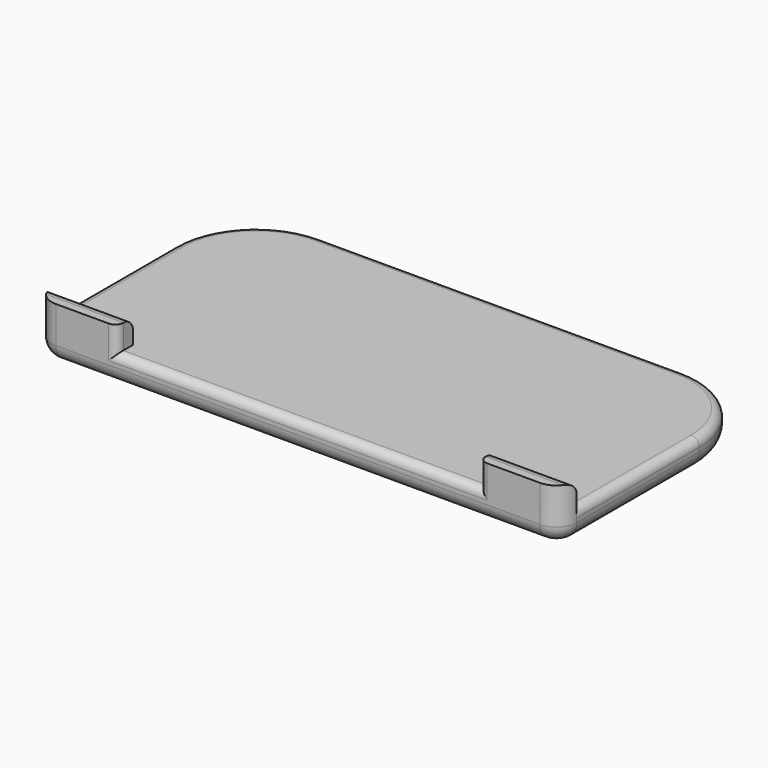
from build123d import *

# Parameters (mm, degrees)
F1_DEPTH    = 8.89
F3_DEPTH    = 7.62
F4_T1_DEPTH = 47.8505725861
F4_T3_DEPTH = 113.1511068404
F4_T6_ANGLE = 90
F4_T8_ANGLE = 90
F5_R        = 5.08
F6_R        = 3.81
F7_R        = 2.54


# Not quite as in the source:
# - a fillet or chamfer that OpenCascade refuses, or shapes differently, is made with other operations: its cross-section is extruded or revolved along the edge and cut away or added


with BuildPart() as f1:
    # F0 (on Top) → F1 (new body)
    with BuildSketch(Plane.XY):
        with BuildLine():
            Line((22.7506106496, 59.7472505152), (-90.4004961908, 59.7472505152))
            ThreePointArc((-90.4004961908, 59.7472505152), (-108.3610084329, 52.3077627574), (-115.8004961908, 34.3472505152))
            Line((-115.8004961908, 34.3472505152), (-115.8004961908, -13.5033220708))
            ThreePointArc((-115.8004961908, -13.5033220708), (-113.9406242513, -17.9934501314), (-109.4504961908, -19.8533220708))
            Line((-109.4504961908, -19.8533220708), (41.8006106496, -19.8533220708))
            ThreePointArc((41.8006106496, -19.8533220708), (46.2907387101, -17.9934501314), (48.1506106496, -13.5033220708))
            Line((48.1506106496, -13.5033220708), (48.1506106496, 34.3472505152))
            ThreePointArc((48.1506106496, 34.3472505152), (40.7111228917, 52.3077627574), (22.7506106496, 59.7472505152))
        make_face()
    extrude(amount=F1_DEPTH)

    # F2 (on face) → F3 (join)
    with BuildSketch(Plane.XY.offset(8.89)):
        with BuildLine():
            ThreePointArc((41.8006106496, -19.8533220708), (46.2907387101, -17.9934501314), (48.1506106496, -13.5033220708))
            Line((48.1506106496, -13.5033220708), (22.7506106496, -13.5033220708))
            Line((22.7506106496, -13.5033220708), (22.7506106496, -19.8533220708))
            Line((22.7506106496, -19.8533220708), (41.8006106496, -19.8533220708))
        make_face()
        with BuildLine():
            Line((-90.4004961908, -13.5033220708), (-115.8004961908, -13.5033220708))
            ThreePointArc((-115.8004961908, -13.5033220708), (-113.9406242513, -17.9934501314), (-109.4504961908, -19.8533220708))
            Line((-109.4504961908, -19.8533220708), (-90.4004961908, -19.8533220708))
            Line((-90.4004961908, -19.8533220708), (-90.4004961908, -13.5033220708))
        make_face()
    extrude(amount=F3_DEPTH)

    # F4: fillet of radius 2.54 on 1 edges, made by hand

    # F4_s2 → F4_t1 (cut)
    with BuildSketch(Plane.XZ.offset(-34.3472505152)):
        with BuildLine():
            ThreePointArc((45.6106106496, 8.89), (47.4066618738, 8.1460512242), (48.1506106496, 6.35))
            Line((48.1506106496, 6.35), (48.1506106496, 8.89))
            Line((48.1506106496, 8.89), (45.6106106496, 8.89))
        make_face()
        with BuildLine():
            ThreePointArc((-113.2604961908, 8.89), (-115.056547415, 8.1460512242), (-115.8004961908, 6.35))
            Line((-115.8004961908, 6.35), (-115.8004961908, 8.89))
            Line((-115.8004961908, 8.89), (-113.2604961908, 8.89))
        make_face()
    extrude(amount=F4_T1_DEPTH, mode=Mode.SUBTRACT)

    # F4_s4 → F4_t3 (cut)
    with BuildSketch(Plane.YZ.offset(-90.4004961908)):
        with BuildLine():
            ThreePointArc((57.2072505152, 8.89), (59.0033017394, 8.1460512242), (59.7472505152, 6.35))
            Line((59.7472505152, 6.35), (59.7472505152, 8.89))
            Line((59.7472505152, 8.89), (57.2072505152, 8.89))
        make_face()
    extrude(amount=F4_T3_DEPTH, mode=Mode.SUBTRACT)

    # F4_s5 → F4_t6 (revolve, cut)
    with BuildSketch(Plane.XZ.offset(-34.3472505152)):
        with BuildLine():
            ThreePointArc((48.1506106496, 6.35), (47.4066618738, 8.1460512242), (45.6106106496, 8.89))
            Line((45.6106106496, 8.89), (48.1506106496, 8.89))
            Line((48.1506106496, 8.89), (48.1506106496, 6.35))
        make_face()
    revolve(axis=Axis((22.7506106496, 34.3472505152, 8.89), (0, 0, 1)), revolution_arc=F4_T6_ANGLE, mode=Mode.SUBTRACT)

    # F4_s7 → F4_t8 (revolve, cut)
    with BuildSketch(Plane.YZ.offset(-90.4004961908)):
        with BuildLine():
            ThreePointArc((57.2072505152, 8.89), (59.0033017394, 8.1460512242), (59.7472505152, 6.35))
            Line((59.7472505152, 6.35), (59.7472505152, 8.89))
            Line((59.7472505152, 8.89), (57.2072505152, 8.89))
        make_face()
    revolve(axis=Axis((-90.4004961908, 34.3472505152, 8.89), (0, 0, 1)), revolution_arc=F4_T8_ANGLE, mode=Mode.SUBTRACT)

    # F5
    f5_edges = [f1.edges().sort_by_distance(p)[0] for p in [
        (-33.824943, 59.747251, 0),
    ]]
    fillet(f5_edges, radius=F5_R)

    # F6
    f6_edges = [f1.edges().sort_by_distance(p)[0] for p in [
        (35.450611, -13.503322, 16.51),
        (-103.100496, -13.503322, 16.51),
    ]]
    fillet(f6_edges, radius=F6_R)

    # F7
    f7_edges = [f1.edges().sort_by_distance(p)[0] for p in [
        (-90.400496, -19.853322, 12.7),
        (-33.824943, -19.853322, 8.89),
        (22.750611, -19.853322, 12.7),
    ]]
    fillet(f7_edges, radius=F7_R)


solid = f1.part
